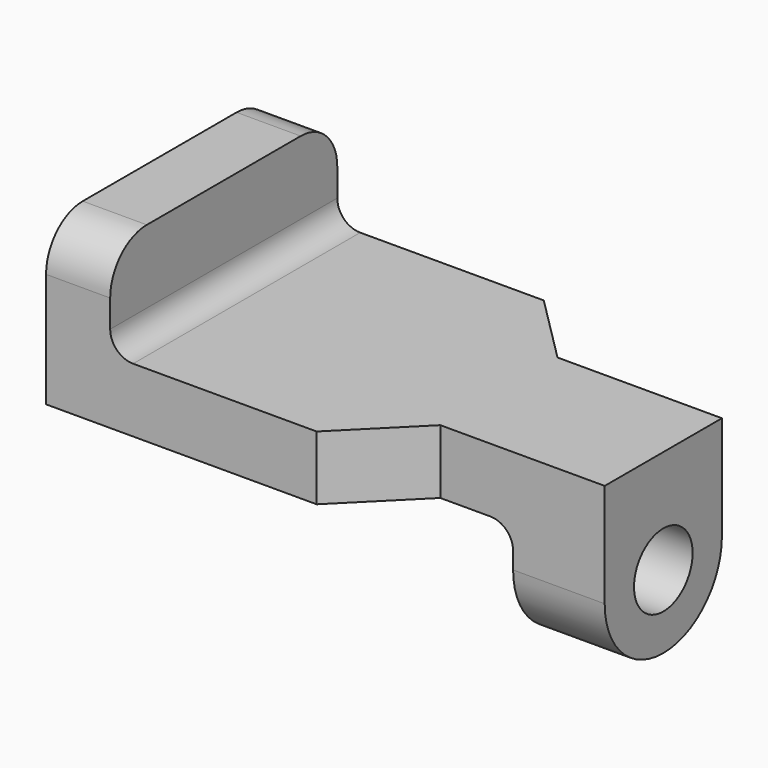
from build123d import *

# Parameters (mm, degrees)
F1_DEPTH = 62
F2_R     = 10
F3_R     = 5
F4_R     = 5
F6_DEPTH = 666
F7_R     = 15.99999
F8_R     = 8
F9_DEPTH = 25


# Not quite as in the source:
# - a fillet or chamfer is up to 0.001 mm smaller than in the source, because OpenCascade refuses the exact size


with BuildPart() as f1:
    # F0 (on Front) → F1 (new body)
    with BuildSketch(Plane.XZ):
        Polygon((-76, 67.66280128), (-90, 67.66280128), (-90, 32.66280128), (0, 32.66280128), (0, 8.0000054104), (20, 8.0000054104), (20, 46.66280128), (-76, 46.66280128), align=None)
    extrude(amount=F1_DEPTH)

    # F2
    f2_edges = [f1.edges().sort_by_distance(p)[0] for p in [
        (-83, -62, 67.662801),
        (-83, 0, 67.662801),
    ]]
    fillet(f2_edges, radius=F2_R)

    # F3
    f3_edges = [f1.edges().sort_by_distance(p)[0] for p in [
        (-76, -31, 46.662801),
    ]]
    fillet(f3_edges, radius=F3_R)

    # F4
    f4_edges = [f1.edges().sort_by_distance(p)[0] for p in [
        (0, -31, 32.662801),
    ]]
    fillet(f4_edges, radius=F4_R)

    # F5 (on face) → F6 (cut)
    with BuildSketch(Plane.XY.offset(46.66280128)):
        Polygon((20, -62), (20, -47), (-15.907, -47), (-30.907, -62), align=None)
        Polygon((-15.907, -15), (20, -15), (20, 0), (-30.907, 0), align=None)
    extrude(amount=-F6_DEPTH, mode=Mode.SUBTRACT)

    # F7 (radius 16 in the source; OpenCascade refuses exactly that, so slightly less here)
    f7_edges = [f1.edges().sort_by_distance(p)[0] for p in [
        (10, -47, 8.000005),
        (10, -15, 8.000005),
    ]]
    fillet(f7_edges, radius=F7_R)

    # F8 (on face) → F9 (cut)
    with BuildSketch(Plane.YZ.offset(20)):
        with Locations((-31, 24.0000054104)):
            Circle(F8_R)
    extrude(amount=-F9_DEPTH, mode=Mode.SUBTRACT)


solid = f1.part
